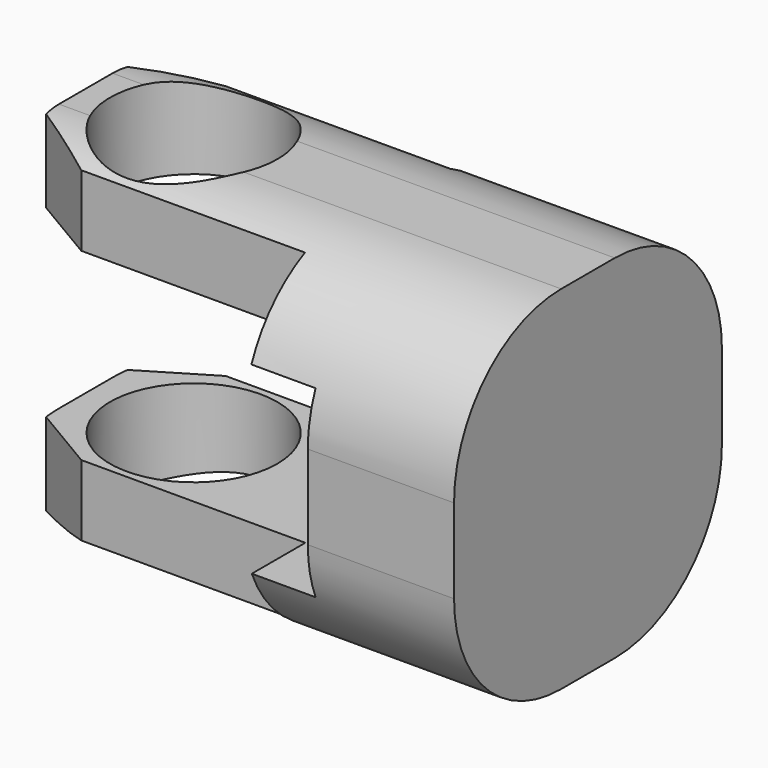
from build123d import *

# Parameters (mm, degrees)
F1_DEPTH    = 25.4
F3_R        = 10.16
F2_R        = 6.35
F4_DEPTH    = 26.7233065934
F6_DEPTH    = 26.7232814104
F7_T1_DEPTH = 66.7645981405
F7_T3_DEPTH = 66.7279267596
F9_DEPTH    = 50.8


# Not quite as in the source:
# - a fillet or chamfer that OpenCascade refuses, or shapes differently, is made with other operations: its cross-section is extruded or revolved along the edge and cut away or added


with BuildPart() as f1:
    # F0 (on Front) → F1 (new body)
    with BuildSketch(Plane.XZ):
        Polygon((27.0092859864, -6.985), (19.05, -6.985), (0, -6.985), (0, -13.335), (38.1, -13.335), (38.1, 13.3873065934), (0, 13.335), (0, 6.985), (19.05, 6.985), (27.0092859864, 6.985), align=None)
    extrude(amount=F1_DEPTH)

    # F3
    f3_edges = [f1.edges().sort_by_distance(p)[0] for p in [
        (0, 0, -10.16),
        (0, 0, 10.16),
        (0, -25.4, 10.16),
        (0, -25.4, -10.16),
    ]]
    fillet(f3_edges, radius=F3_R)

    # F2 (on face) → F4 (cut, through all)
    with BuildSketch(Plane(origin=(0, 0, -13.335), x_dir=(1, 0, 0), z_dir=(0, 0, -1))):
        with Locations((8.1856111065, 12.7)):
            Circle(F2_R)
    extrude(amount=-F4_DEPTH, mode=Mode.SUBTRACT)

    # F5 (on face) → F6 (cut, through all)
    with BuildSketch(Plane(origin=(-0.0183072732, 0, 13.3349748664), x_dir=(0.9999990576, 0, 0.0013728752), z_dir=(-0.0013728752, 0, 0.9999990576))):
        with BuildLine():
            Line((20.423270762, 6.0135265812), (-7.3266747168, -5.8177547927))
            Line((-7.3266747168, -5.8177547927), (0.9929662687, -5.8177547927))
            add(Edge.make_bspline(
                [(10.1783168652, 0), (3.7432331436, 0), (0.9929662687, -5.8177547927)],
                knots=[4.7123889804, 4.7123889804, 4.7123889804, 5.8269772874, 5.8269772874, 5.8269772874], degree=2, weights=[1, 0.792172065, 0.879280631]))
            Line((10.1783168652, 0), (22.1537450551, 0))
            Line((22.1537450551, 0), (20.423270762, 6.0135265812))
        make_face()
        with BuildLine():
            add(Edge.make_bspline(
                [(10.1783168652, 0), (3.7432331436, 0), (0.9929662687, -5.8177547927)],
                knots=[4.7123889804, 4.7123889804, 4.7123889804, 5.8269772874, 5.8269772874, 5.8269772874], degree=2, weights=[1, 0.792172065, 0.879280631]))
            Line((0.9929662687, -5.8177547927), (22.1537450551, -5.8177547927))
            Line((22.1537450551, -5.8177547927), (22.1537450551, 0))
            Line((22.1537450551, 0), (10.1783168652, 0))
        make_face()
        with BuildLine():
            Line((22.1537450551, -25.4), (22.1537450551, -19.5822452073))
            Line((22.1537450551, -19.5822452073), (0.9929662687, -19.5822452073))
            add(Edge.make_bspline(
                [(0.9929662687, -19.5822452073), (3.7432331436, -25.4), (10.1783168652, -25.4)],
                knots=[0.4562080198, 0.4562080198, 0.4562080198, 1.5707963268, 1.5707963268, 1.5707963268], degree=2, weights=[0.879280631, 0.792172065, 1]))
            Line((10.1783168652, -25.4), (22.1537450551, -25.4))
        make_face()
        with BuildLine():
            Line((0.9929662687, -19.5822452073), (-6.3022147662, -19.5822452073))
            Line((-6.3022147662, -19.5822452073), (17.9763548076, -30.6573584676))
            Line((17.9763548076, -30.6573584676), (22.1537450551, -25.4))
            Line((22.1537450551, -25.4), (10.1783168652, -25.4))
            add(Edge.make_bspline(
                [(0.9929662687, -19.5822452073), (3.7432331436, -25.4), (10.1783168652, -25.4)],
                knots=[0.4562080198, 0.4562080198, 0.4562080198, 1.5707963268, 1.5707963268, 1.5707963268], degree=2, weights=[0.879280631, 0.792172065, 1]))
        make_face()
    extrude(amount=-F6_DEPTH, mode=Mode.SUBTRACT)

    # F7: fillet of radius 10.16 on 4 edges, made by hand

    # F7_s2 → F7_t1 (cut)
    with BuildSketch(Plane(origin=(63.5182833364, 0, 0.0872027564), x_dir=(0, 1, 0), z_dir=(-0.9999990576, 0, -0.0013728752))):
        with BuildLine():
            ThreePointArc((-25.4, -3.1749874332), (-22.4242048969, -10.35919233), (-15.24, -13.3349874332))
            Line((-15.24, -13.3349874332), (-25.4, -13.3349874332))
            Line((-25.4, -13.3349874332), (-25.4, -3.1749874332))
        make_face()
        with BuildLine():
            ThreePointArc((0, -3.1749874332), (-2.9757951031, -10.35919233), (-10.16, -13.3349874332))
            Line((-10.16, -13.3349874332), (0, -13.3349874332))
            Line((0, -13.3349874332), (0, -3.1749874332))
        make_face()
    extrude(amount=F7_T1_DEPTH, mode=Mode.SUBTRACT)

    # F7_s4 → F7_t3 (cut)
    with BuildSketch(Plane.YZ.offset(-3.2279267596)):
        with BuildLine():
            ThreePointArc((0, -3.175), (-2.9757951031, -10.3592048969), (-10.16, -13.335))
            Line((-10.16, -13.335), (0, -13.335))
            Line((0, -13.335), (0, -3.175))
        make_face()
        with BuildLine():
            ThreePointArc((-25.4, -3.175), (-22.4242048969, -10.3592048969), (-15.24, -13.335))
            Line((-15.24, -13.335), (-25.4, -13.335))
            Line((-25.4, -13.335), (-25.4, -3.175))
        make_face()
    extrude(amount=F7_T3_DEPTH, mode=Mode.SUBTRACT)

    # F8 (on Top) → F9 (cut, symmetric)
    with BuildSketch(Plane.XY):
        Polygon((-2.6969234459, -10.516657494), (6.3479291275, -5.0737368874), (-5.7385554537, -5.0737368874), (-5.7385554537, -20.2818978578), (6.3479291275, -20.2818978578), (-2.6969234459, -14.9190193042), align=None)
    extrude(amount=F9_DEPTH, both=True, mode=Mode.SUBTRACT)


solid = f1.part
